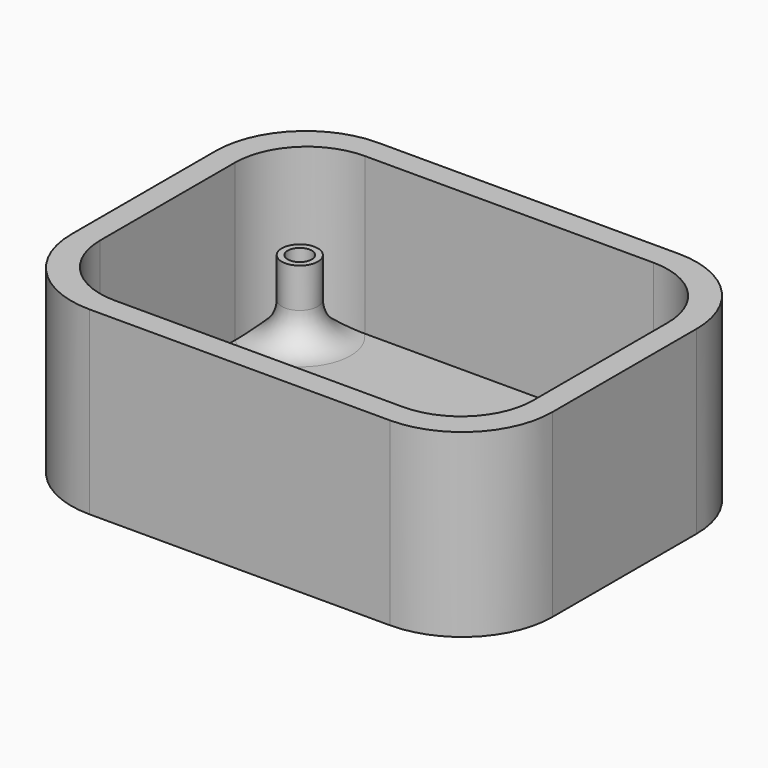
from build123d import *

# Parameters (mm, degrees)
F0_W         = 80
F0_H         = 60
F0_W_2       = 72
F0_H_2       = 52
F0_R         = 3
F0_R_2       = 2
F1_DEPTH     = 4
F2_DEPTH     = 30
F3_DEPTH     = 16
F5_R         = 12
F6_R         = 15
F7_S5_R      = 12
F7_T6_DEPTH  = 15
F7_S11_R     = 12
F7_T12_DEPTH = 15
F7_S17_R     = 12
F7_T18_DEPTH = 15
F7_S23_R     = 12
F7_T24_DEPTH = 15


# Not quite as in the source:
# - a fillet or chamfer that OpenCascade refuses, or shapes differently, is made with other operations: its cross-section is extruded or revolved along the edge and cut away or added


with BuildPart() as f1:
    # F0 (on Top) → F1 (new body)
    with BuildSketch(Plane.XY):
        Rectangle(F0_W, F0_H)
        Rectangle(F0_W_2, F0_H_2, mode=Mode.SUBTRACT)
        Rectangle(F0_W_2, F0_H_2)
        with Locations((-30, -20)):
            Circle(F0_R, mode=Mode.SUBTRACT)
        with Locations((30, -20)):
            Circle(F0_R, mode=Mode.SUBTRACT)
        with Locations((-30, 20)):
            Circle(F0_R, mode=Mode.SUBTRACT)
        with Locations((30, 20)):
            Circle(F0_R, mode=Mode.SUBTRACT)
        with Locations((-30, 20)):
            Circle(F0_R)
        with Locations((-30, 20)):
            Circle(F0_R_2, mode=Mode.SUBTRACT)
        with Locations((30, 20)):
            Circle(F0_R)
        with Locations((30, 20)):
            Circle(F0_R_2, mode=Mode.SUBTRACT)
        with Locations((30, -20)):
            Circle(F0_R)
        with Locations((30, -20)):
            Circle(F0_R_2, mode=Mode.SUBTRACT)
        with Locations((-30, -20)):
            Circle(F0_R)
        with Locations((-30, -20)):
            Circle(F0_R_2, mode=Mode.SUBTRACT)
    extrude(amount=F1_DEPTH)

    # F0 (on Top) → F2 (join)
    with BuildSketch(Plane.XY):
        Rectangle(F0_W, F0_H)
        Rectangle(F0_W_2, F0_H_2, mode=Mode.SUBTRACT)
    extrude(amount=F2_DEPTH)

    # F0 (on Top) → F3 (join)
    with BuildSketch(Plane.XY):
        with Locations((-30, 20)):
            Circle(F0_R)
        with Locations((-30, 20)):
            Circle(F0_R_2, mode=Mode.SUBTRACT)
        with Locations((-30, -20)):
            Circle(F0_R)
        with Locations((-30, -20)):
            Circle(F0_R_2, mode=Mode.SUBTRACT)
        with Locations((30, 20)):
            Circle(F0_R)
        with Locations((30, 20)):
            Circle(F0_R_2, mode=Mode.SUBTRACT)
        with Locations((30, -20)):
            Circle(F0_R)
        with Locations((30, -20)):
            Circle(F0_R_2, mode=Mode.SUBTRACT)
    extrude(amount=F3_DEPTH)

    # F4: union 

    # F5
    f5_edges = [f1.edges().sort_by_distance(p)[0] for p in [
        (-36, 26, 17),
        (36, 26, 17),
        (-36, -26, 17),
        (36, -26, 17),
    ]]
    fillet(f5_edges, radius=F5_R)

    # F6
    f6_edges = [f1.edges().sort_by_distance(p)[0] for p in [
        (40, -30, 15),
        (-40, -30, 15),
        (40, 30, 15),
        (-40, 30, 15),
    ]]
    fillet(f6_edges, radius=F6_R)

    # F7: fillet of radius 5.5 on 4 edges, made by hand


with BuildPart() as f7_tool2:
    # F7_s3 → F7_t4 (revolve)
    with BuildSketch(Plane.XZ.offset(-20)):
        with BuildLine():
            ThreePointArc((-21.4990343146, 3.9996), (-25.3890872965, 5.6109127035), (-27.0004, 9.5009656854))
            Line((-27.0004, 9.5009656854), (-27.5505365685, 9.5009656854))
            ThreePointArc((-27.5505365685, 9.5009656854), (-27.5501365685, 6.7504828427), (-27.5501365685, 4))
            Line((-27.5501365685, 4), (-27, 3.4498634315))
            ThreePointArc((-27, 3.4498634315), (-24.2495171573, 3.4498634315), (-21.4990343146, 3.4494634315))
            Line((-21.4990343146, 3.4494634315), (-21.4990343146, 3.9996))
        make_face()
    revolve(axis=Axis((-30, 20, 4), (0, 0, -1)))

    # F7_s5 → F7_t6 (intersect, symmetric)
    with BuildSketch(Plane.XY.offset(8.4)):
        with Locations((-24, 14)):
            Circle(F7_S5_R)
    extrude(amount=F7_T6_DEPTH, both=True, mode=Mode.INTERSECT)


with BuildPart() as f1_1:
    add(f1.part)

    # F7_t1: union F7_tool2
    add(f7_tool2.part)


with BuildPart() as f7_tool8:
    # F7_s9 → F7_t10 (revolve)
    with BuildSketch(Plane.XZ.offset(20)):
        with BuildLine():
            ThreePointArc((-21.4990343146, 3.9996), (-25.3890872965, 5.6109127035), (-27.0004, 9.5009656854))
            Line((-27.0004, 9.5009656854), (-27.5505365685, 9.5009656854))
            ThreePointArc((-27.5505365685, 9.5009656854), (-27.5501365685, 6.7504828427), (-27.5501365685, 4))
            Line((-27.5501365685, 4), (-27, 3.4498634315))
            ThreePointArc((-27, 3.4498634315), (-24.2495171573, 3.4498634315), (-21.4990343146, 3.4494634315))
            Line((-21.4990343146, 3.4494634315), (-21.4990343146, 3.9996))
        make_face()
    revolve(axis=Axis((-30, -20, 4), (0, 0, -1)))

    # F7_s11 → F7_t12 (intersect, symmetric)
    with BuildSketch(Plane.XY.offset(8.4)):
        with Locations((-24, -14)):
            Circle(F7_S11_R)
    extrude(amount=F7_T12_DEPTH, both=True, mode=Mode.INTERSECT)


with BuildPart() as f1_2:
    add(f1_1.part)

    # F7_t7: union F7_tool8
    add(f7_tool8.part)


with BuildPart() as f7_tool14:
    # F7_s15 → F7_t16 (revolve)
    with BuildSketch(Plane.XZ.offset(-20)):
        with BuildLine():
            ThreePointArc((38.5009656854, 3.9996), (34.6109127035, 5.6109127035), (32.9996, 9.5009656854))
            Line((32.9996, 9.5009656854), (32.4494634315, 9.5009656854))
            ThreePointArc((32.4494634315, 9.5009656854), (32.4498634315, 6.7504828427), (32.4498634315, 4))
            Line((32.4498634315, 4), (33, 3.4498634315))
            ThreePointArc((33, 3.4498634315), (35.7504828427, 3.4498634315), (38.5009656854, 3.4494634315))
            Line((38.5009656854, 3.4494634315), (38.5009656854, 3.9996))
        make_face()
    revolve(axis=Axis((30, 20, 4), (0, 0, -1)))

    # F7_s17 → F7_t18 (intersect, symmetric)
    with BuildSketch(Plane.XY.offset(8.4)):
        with Locations((24, 14)):
            Circle(F7_S17_R)
    extrude(amount=F7_T18_DEPTH, both=True, mode=Mode.INTERSECT)


with BuildPart() as f1_3:
    add(f1_2.part)

    # F7_t13: union F7_tool14
    add(f7_tool14.part)


with BuildPart() as f7_tool20:
    # F7_s21 → F7_t22 (revolve)
    with BuildSketch(Plane.XZ.offset(20)):
        with BuildLine():
            ThreePointArc((38.5009656854, 3.9996), (34.6109127035, 5.6109127035), (32.9996, 9.5009656854))
            Line((32.9996, 9.5009656854), (32.4494634315, 9.5009656854))
            ThreePointArc((32.4494634315, 9.5009656854), (32.4498634315, 6.7504828427), (32.4498634315, 4))
            Line((32.4498634315, 4), (33, 3.4498634315))
            ThreePointArc((33, 3.4498634315), (35.7504828427, 3.4498634315), (38.5009656854, 3.4494634315))
            Line((38.5009656854, 3.4494634315), (38.5009656854, 3.9996))
        make_face()
    revolve(axis=Axis((30, -20, 4), (0, 0, -1)))

    # F7_s23 → F7_t24 (intersect, symmetric)
    with BuildSketch(Plane.XY.offset(8.4)):
        with Locations((24, -14)):
            Circle(F7_S23_R)
    extrude(amount=F7_T24_DEPTH, both=True, mode=Mode.INTERSECT)


with BuildPart() as f1_4:
    add(f1_3.part)

    # F7_t19: union F7_tool20
    add(f7_tool20.part)


solid = f1_4.part
